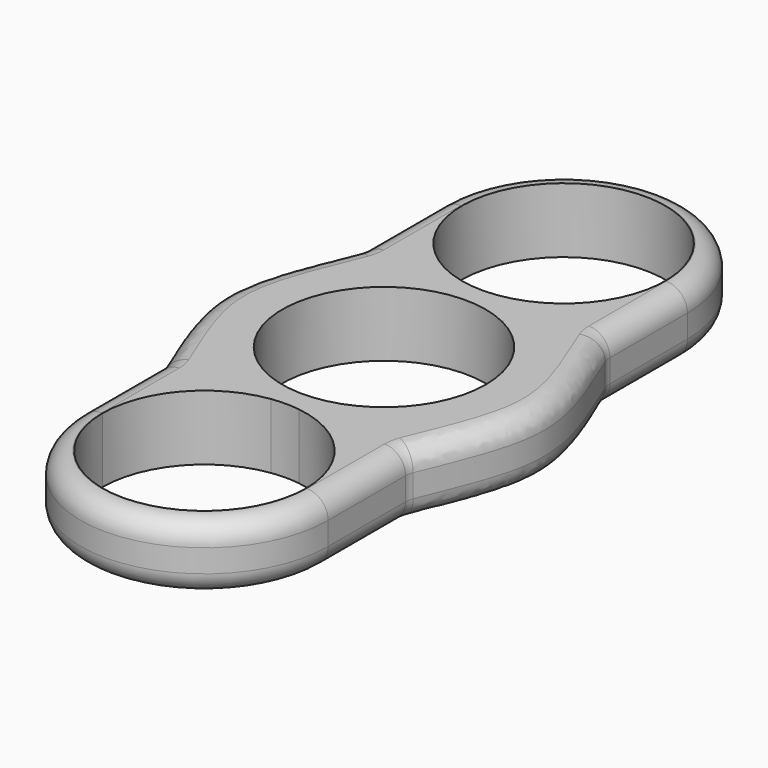
from build123d import *

# Parameters (mm, degrees)
F0_R     = 11.1
F1_DEPTH = 7.1
F2_R     = 2.3


with BuildPart() as f1:
    # F0 (on Top) → F1 (new body)
    with BuildSketch(Plane.XY):
        with BuildLine():
            Line((11.1, 24.4949632536), (13.5, 24.4949632536))
            ThreePointArc((13.5, 24.4949632536), (0, 37.9949632536), (-13.5, 24.4949632536))
            Line((-13.5, 24.4949632536), (-11.1, 24.4949632536))
            ThreePointArc((-11.1, 24.4949632536), (0, 35.5949632536), (11.1, 24.4949632536))
        make_face()
        with BuildLine():
            Line((-13.5, 13.5), (-1.5234116489, 13.5))
            ThreePointArc((-1.5234116489, 13.5), (-8.3701812795, 17.2045541191), (-11.1, 24.4949632536))
            Line((-11.1, 24.4949632536), (-13.5, 24.4949632536))
            Line((-13.5, 24.4949632536), (-13.5, 13.5))
        make_face()
        with BuildLine():
            Line((1.5234116489, 13.5), (13.5, 13.5))
            Line((13.5, 13.5), (13.5, 24.4949632536))
            Line((13.5, 24.4949632536), (11.1, 24.4949632536))
            ThreePointArc((11.1, 24.4949632536), (8.3701812795, 17.2045541191), (1.5234116489, 13.5))
        make_face()
        with BuildLine():
            Line((13.5, -13.5), (13.5, 13.5))
            Line((13.5, 13.5), (1.5234116489, 13.5))
            ThreePointArc((1.5234116489, 13.5), (0, 13.3949632536), (-1.5234116489, 13.5))
            Line((-1.5234116489, 13.5), (-13.5, 13.5))
            Line((-13.5, 13.5), (-13.5, -13.5))
            Line((-13.5, -13.5), (-1.5048250316, -13.5))
            ThreePointArc((-1.5048250316, -13.5), (0, -13.3975225221), (1.5048250316, -13.5))
            Line((1.5048250316, -13.5), (13.5, -13.5))
        make_face()
        Circle(F0_R, mode=Mode.SUBTRACT)
        with BuildLine():
            add(Edge.make_bspline(
                [(13.5, 13.5), (15.2430341691, 9), (19.7569658309, 0), (15.2430341691, -9), (13.5, -13.5)],
                knots=[0, 0, 0, 0, 0.5, 1, 1, 1, 1], degree=3))
            Line((13.5, 13.5), (13.5, -13.5))
        make_face()
        with BuildLine():
            Line((-13.5, -13.5), (-13.5, 13.5))
            add(Edge.make_bspline(
                [(-13.5, 13.5), (-15.2435445338, 9), (-19.7564554662, 0), (-15.2435445338, -9), (-13.5, -13.5)],
                knots=[0, 0, 0, 0, 0.5, 1, 1, 1, 1], degree=3))
        make_face()
        with BuildLine():
            ThreePointArc((-11.1, -24.4975225221), (-8.3640169133, -17.2000420614), (-1.5048250316, -13.5))
            Line((-1.5048250316, -13.5), (-13.5, -13.5))
            Line((-13.5, -13.5), (-13.5, -24.4975225221))
            Line((-13.5, -24.4975225221), (-11.1, -24.4975225221))
        make_face()
        with BuildLine():
            Line((13.5, -24.4975225221), (13.5, -13.5))
            Line((13.5, -13.5), (1.5048250316, -13.5))
            ThreePointArc((1.5048250316, -13.5), (8.3640169133, -17.2000420614), (11.1, -24.4975225221))
            Line((11.1, -24.4975225221), (13.5, -24.4975225221))
        make_face()
        with BuildLine():
            ThreePointArc((-13.5, -24.4975225221), (0, -37.9975225221), (13.5, -24.4975225221))
            Line((13.5, -24.4975225221), (11.1, -24.4975225221))
            ThreePointArc((11.1, -24.4975225221), (0, -35.5975225221), (-11.1, -24.4975225221))
            Line((-11.1, -24.4975225221), (-13.5, -24.4975225221))
        make_face()
    extrude(amount=F1_DEPTH)

    # F2
    f2_edges = [f1.edges().sort_by_distance(p)[0] for p in [
        (13.5, -13.5, 3.55),
        (17.5, 0, 7.1),
        (17.5, 0, 0),
        (13.5, 13.5, 3.55),
        (13.5, 18.997482, 7.1),
        (0, 37.994963, 7.1),
        (0, 37.994963, 0),
        (13.5, 24.494963, 3.55),
        (13.5, 18.997482, 0),
        (-13.5, 18.997482, 7.1),
        (-17.5, 0, 7.1),
        (0, -37.997523, 7.1),
        (-13.5, -18.998761, 7.1),
        (13.5, -18.998761, 7.1),
        (13.5, -18.998761, 0),
        (0, -37.997523, 0),
        (-13.5, -13.5, 3.55),
        (-13.5, 13.5, 3.55),
        (-13.5, 18.997482, 0),
        (-17.5, 0, 0),
        (-13.5, -18.998761, 0),
    ]]
    fillet(f2_edges, radius=F2_R)


solid = f1.part
